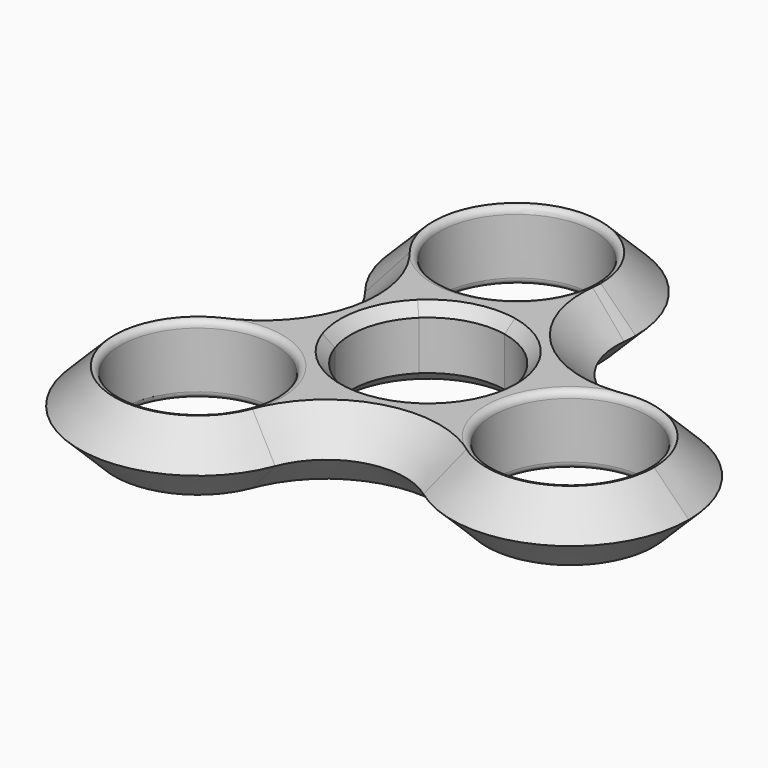
from build123d import *

# Parameters (mm, degrees)
F0_R     = 11.1
F1_DEPTH = 10
F2_SIZE  = 4.99999
F4_SIZE  = 1.5


# Not quite as in the source:
# - a fillet or chamfer that OpenCascade refuses, or shapes differently, is made with other operations: its cross-section is extruded or revolved along the edge and cut away or added
# - a fillet or chamfer is up to 0.001 mm smaller than in the source, because OpenCascade refuses the exact size


with BuildPart() as f1:
    # F0 (on Top) → F1 (new body)
    with BuildSketch(Plane.XY):
        with BuildLine():
            ThreePointArc((-8.9008040787, 8.0483344086), (-3.3470312857, 11.5237746235), (3.2044142943, 11.5642435563))
            ThreePointArc((3.2044142943, 11.5642435563), (7.5784009732, 16.6578149501), (9.6392593011, 23.047579575))
            ThreePointArc((9.6392593011, 23.047579575), (9.7208671752, 24.0063382249), (9.7480988809, 24.9681783508))
            ThreePointArc((9.7480988809, 24.9681783508), (-12.909602396, 40.9990989813), (-20.4860677382, 14.297806572))
            ThreePointArc((-20.4860677382, 14.297806572), (-15.3228623754, 10.0062404951), (-8.9008040787, 8.0483344086))
        make_face()
        with Locations((-7.2519011191, 24.9681783508)):
            Circle(F0_R, mode=Mode.SUBTRACT)
        with BuildLine():
            ThreePointArc((3.2044142943, 11.5642435563), (8.2952723159, 8.6711277931), (11.410994073, 3.7133831296))
            ThreePointArc((11.410994073, 3.7133831296), (16.3058703698, 8.3086431928), (22.5981031738, 10.6504449244))
            ThreePointArc((22.5981031738, 10.6504449244), (13.0446528896, 13.6357009046), (9.6392593011, 23.047579575))
            ThreePointArc((9.6392593011, 23.047579575), (7.5784009732, 16.6578149501), (3.2044142943, 11.5642435563))
        make_face()
        with BuildLine():
            ThreePointArc((22.5981031738, 10.6504449244), (16.3058703698, 8.3086431928), (11.410994073, 3.7133831296))
            ThreePointArc((11.410994073, 3.7133831296), (11.8518338006, 1.8799030726), (12, 0))
            ThreePointArc((12, 0), (11.07283247, -4.6251898438), (8.4346031515, -8.5356587137))
            ThreePointArc((8.4346031515, -8.5356587137), (10.6749837374, -14.8647126588), (15.1909877347, -19.8328045366))
            ThreePointArc((15.1909877347, -19.8328045366), (32.9376604929, -21.3090514083), (42.264828105, -6.139092834))
            ThreePointArc((42.264828105, -6.139092834), (36.302619464, 6.7902212203), (22.5981031738, 10.6504449244))
        make_face()
        with Locations((25.264828105, -6.139092834)):
            Circle(F0_R, mode=Mode.SUBTRACT)
        with BuildLine():
            ThreePointArc((15.1909877347, -19.8328045366), (10.6749837374, -14.8647126588), (8.4346031515, -8.5356587137))
            ThreePointArc((8.4346031515, -8.5356587137), (3.3912632474, -11.5108354861), (-2.459549488, -11.7452380272))
            ThreePointArc((-2.459549488, -11.7452380272), (-1.295062841, -15.2163673164), (-0.9008049677, -18.8563300117))
            ThreePointArc((-0.9008049677, -18.8563300117), (-1.1808473044, -21.9292790409), (-2.0117479955, -24.9009862083))
            ThreePointArc((-2.0117479955, -24.9009862083), (5.3328992991, -18.1012566756), (15.1909877347, -19.8328045366))
        make_face()
        with BuildLine():
            ThreePointArc((-0.9008049677, -18.8563300117), (-1.295062841, -15.2163673164), (-2.459549488, -11.7452380272))
            ThreePointArc((-2.459549488, -11.7452380272), (-8.2619099851, -8.7029215438), (-11.6015857751, -3.0664649849))
            ThreePointArc((-11.6015857751, -3.0664649849), (-18.2060105223, -1.859069951), (-24.7628314098, -3.3027904432))
            ThreePointArc((-24.7628314098, -3.3027904432), (-29.6051774466, -31.1854688655), (-2.0117479955, -24.9009862083))
            ThreePointArc((-2.0117479955, -24.9009862083), (-1.1808473044, -21.9292790409), (-0.9008049677, -18.8563300117))
        make_face()
        with Locations((-17.9008049677, -18.8563300117)):
            Circle(F0_R, mode=Mode.SUBTRACT)
        with BuildLine():
            ThreePointArc((-11.6015857751, -3.0664649849), (-11.6606898946, 2.8334274618), (-8.9008040787, 8.0483344086))
            ThreePointArc((-8.9008040787, 8.0483344086), (-15.3228623754, 10.0062404951), (-20.4860677382, 14.297806572))
            ThreePointArc((-20.4860677382, 14.297806572), (-18.2811908203, 4.4421409517), (-24.7628314098, -3.3027904432))
            ThreePointArc((-24.7628314098, -3.3027904432), (-18.2060105223, -1.859069951), (-11.6015857751, -3.0664649849))
        make_face()
        with BuildLine():
            ThreePointArc((-7.7210685302, 7.9746536446), (-3.0960039393, 10.6594915267), (2.2477068882, 10.8700420305))
            ThreePointArc((2.2477068882, 10.8700420305), (2.732096018, 11.208825126), (3.2044142943, 11.5642435563))
            ThreePointArc((3.2044142943, 11.5642435563), (-3.3470312857, 11.5237746235), (-8.9008040787, 8.0483344086))
            ThreePointArc((-8.9008040787, 8.0483344086), (-8.3115768891, 8.0012373401), (-7.7210685302, 7.9746536446))
        make_face()
        with BuildLine():
            ThreePointArc((-10.5195848427, -3.5423628749), (-10.7861381525, 2.6209204022), (-7.7210685302, 7.9746536446))
            ThreePointArc((-7.7210685302, 7.9746536446), (-8.3115768891, 8.0012373401), (-8.9008040787, 8.0483344086))
            ThreePointArc((-8.9008040787, 8.0483344086), (-11.6606898946, 2.8334274618), (-11.6015857751, -3.0664649849))
            ThreePointArc((-11.6015857751, -3.0664649849), (-11.0564478261, -3.2950069536), (-10.5195848427, -3.5423628749))
        make_face()
        with BuildLine():
            ThreePointArc((2.2477068882, 10.8700420305), (7.6731268923, 8.0207932086), (10.759840528, 2.7268721665))
            ThreePointArc((10.759840528, 2.7268721665), (11.0768405192, 3.2257888132), (11.410994073, 3.7133831296))
            ThreePointArc((11.410994073, 3.7133831296), (8.2952723159, 8.6711277931), (3.2044142943, 11.5642435563))
            ThreePointArc((3.2044142943, 11.5642435563), (2.732096018, 11.208825126), (2.2477068882, 10.8700420305))
        make_face()
        with BuildLine():
            ThreePointArc((10.759840528, 2.7268721665), (11.0146318563, 1.3740033005), (11.1, 0))
            ThreePointArc((11.1, 0), (10.3787556413, -3.9359155654), (8.3087511103, -7.3603434015))
            ThreePointArc((8.3087511103, -7.3603434015), (8.3614588742, -7.9490952222), (8.4346031515, -8.5356587137))
            ThreePointArc((8.4346031515, -8.5356587137), (11.07283247, -4.6251898438), (12, 0))
            ThreePointArc((12, 0), (11.8518338006, 1.8799030726), (11.410994073, 3.7133831296))
            ThreePointArc((11.410994073, 3.7133831296), (11.0768405192, 3.2257888132), (10.759840528, 2.7268721665))
        make_face()
        with BuildLine():
            ThreePointArc((8.4346031515, -8.5356587137), (8.3614588742, -7.9490952222), (8.3087511103, -7.3603434015))
            ThreePointArc((8.3087511103, -7.3603434015), (3.1369185038, -10.6475228246), (-2.9910212262, -10.6894243074))
            ThreePointArc((-2.9910212262, -10.6894243074), (-2.7161060538, -11.2127105225), (-2.459549488, -11.7452380272))
            ThreePointArc((-2.459549488, -11.7452380272), (3.3912632474, -11.5108354861), (8.4346031515, -8.5356587137))
        make_face()
        with BuildLine():
            ThreePointArc((-2.459549488, -11.7452380272), (-2.7161060538, -11.2127105225), (-2.9910212262, -10.6894243074))
            ThreePointArc((-2.9910212262, -10.6894243074), (-7.6422667362, -8.0502024281), (-10.5195848427, -3.5423628749))
            ThreePointArc((-10.5195848427, -3.5423628749), (-11.0564478261, -3.2950069536), (-11.6015857751, -3.0664649849))
            ThreePointArc((-11.6015857751, -3.0664649849), (-8.2619099851, -8.7029215438), (-2.459549488, -11.7452380272))
        make_face()
    extrude(amount=F1_DEPTH)

    # F2 (size 5 in the source; OpenCascade refuses exactly that, so slightly less here)
    f2_edges = [f1.edges().sort_by_distance(p)[0] for p in [
        (-29.605177, -31.185469, 10),
        (41.784139, -10.153115, 0),
    ]]
    chamfer(f2_edges, length=F2_SIZE)

    # F3: fillet of radius 1 on 6 edges, made by hand

    # F3_s1 → F3_t2 (revolve, cut)
    with BuildSketch(Plane.XZ.offset(6.139092834)):
        with BuildLine():
            ThreePointArc((37.364728105, 10.0001), (36.6576213238, 9.7072067812), (36.364728105, 9.0001))
            Line((36.364728105, 9.0001), (36.344728105, 9.0001))
            ThreePointArc((36.344728105, 9.0001), (36.344828105, 9.50005), (36.344828105, 10))
            Line((36.344828105, 10), (36.364828105, 10.02))
            ThreePointArc((36.364828105, 10.02), (36.864778105, 10.02), (37.364728105, 10.0201))
            Line((37.364728105, 10.0201), (37.364728105, 10.0001))
        make_face()
    revolve(axis=Axis((25.264828105, -6.139092834, 10), (0, 0, 1)), mode=Mode.SUBTRACT)

    # F3_s3 → F3_t4 (revolve, cut)
    with BuildSketch(Plane.XZ.offset(-24.9681783508)):
        with BuildLine():
            ThreePointArc((4.8479988809, 10.0001), (4.1408920997, 9.7072067812), (3.8479988809, 9.0001))
            Line((3.8479988809, 9.0001), (3.8279988809, 9.0001))
            ThreePointArc((3.8279988809, 9.0001), (3.8280988809, 9.50005), (3.8280988809, 10))
            Line((3.8280988809, 10), (3.8480988809, 10.02))
            ThreePointArc((3.8480988809, 10.02), (4.3480488809, 10.02), (4.8479988809, 10.0201))
            Line((4.8479988809, 10.0201), (4.8479988809, 10.0001))
        make_face()
    revolve(axis=Axis((-7.2519011191, 24.9681783508, 10), (0, 0, 1)), mode=Mode.SUBTRACT)

    # F3_s5 → F3_t6 (revolve, cut)
    with BuildSketch(Plane.XZ.offset(18.8563300117)):
        with BuildLine():
            ThreePointArc((-5.8009049677, 10.0001), (-6.5080117489, 9.7072067812), (-6.8009049677, 9.0001))
            Line((-6.8009049677, 9.0001), (-6.8209049677, 9.0001))
            ThreePointArc((-6.8209049677, 9.0001), (-6.8208049677, 9.50005), (-6.8208049677, 10))
            Line((-6.8208049677, 10), (-6.8008049677, 10.02))
            ThreePointArc((-6.8008049677, 10.02), (-6.3008549677, 10.02), (-5.8009049677, 10.0201))
            Line((-5.8009049677, 10.0201), (-5.8009049677, 10.0001))
        make_face()
    revolve(axis=Axis((-17.9008049677, -18.8563300117, 10), (0, 0, 1)), mode=Mode.SUBTRACT)

    # F3_s7 → F3_t8 (revolve, cut)
    with BuildSketch(Plane.XZ.offset(6.139092834)):
        with BuildLine():
            ThreePointArc((37.364728105, -0.0001), (36.6576213238, 0.2927932188), (36.364728105, 0.9999))
            Line((36.364728105, 0.9999), (36.344728105, 0.9999))
            ThreePointArc((36.344728105, 0.9999), (36.344828105, 0.49995), (36.344828105, 0))
            Line((36.344828105, 0), (36.364828105, -0.02))
            ThreePointArc((36.364828105, -0.02), (36.864778105, -0.02), (37.364728105, -0.0201))
            Line((37.364728105, -0.0201), (37.364728105, -0.0001))
        make_face()
    revolve(axis=Axis((25.264828105, -6.139092834, 0), (0, 0, 1)), mode=Mode.SUBTRACT)

    # F3_s9 → F3_t10 (revolve, cut)
    with BuildSketch(Plane.XZ.offset(-24.9681783508)):
        with BuildLine():
            ThreePointArc((4.8479988809, -0.0001), (4.1408920997, 0.2927932188), (3.8479988809, 0.9999))
            Line((3.8479988809, 0.9999), (3.8279988809, 0.9999))
            ThreePointArc((3.8279988809, 0.9999), (3.8280988809, 0.49995), (3.8280988809, 0))
            Line((3.8280988809, 0), (3.8480988809, -0.02))
            ThreePointArc((3.8480988809, -0.02), (4.3480488809, -0.02), (4.8479988809, -0.0201))
            Line((4.8479988809, -0.0201), (4.8479988809, -0.0001))
        make_face()
    revolve(axis=Axis((-7.2519011191, 24.9681783508, 0), (0, 0, 1)), mode=Mode.SUBTRACT)

    # F3_s11 → F3_t12 (revolve, cut)
    with BuildSketch(Plane.XZ.offset(18.8563300117)):
        with BuildLine():
            ThreePointArc((-5.8009049677, -0.0001), (-6.5080117489, 0.2927932188), (-6.8009049677, 0.9999))
            Line((-6.8009049677, 0.9999), (-6.8209049677, 0.9999))
            ThreePointArc((-6.8209049677, 0.9999), (-6.8208049677, 0.49995), (-6.8208049677, 0))
            Line((-6.8208049677, 0), (-6.8008049677, -0.02))
            ThreePointArc((-6.8008049677, -0.02), (-6.3008549677, -0.02), (-5.8009049677, -0.0201))
            Line((-5.8009049677, -0.0201), (-5.8009049677, -0.0001))
        make_face()
    revolve(axis=Axis((-17.9008049677, -18.8563300117, 0), (0, 0, 1)), mode=Mode.SUBTRACT)

    # F4
    f4_edges = [f1.edges().sort_by_distance(p)[0] for p in [
        (2.991021, 10.689424, 0),
        (-2.991021, -10.689424, 5),
        (2.991021, 10.689424, 10),
    ]]
    chamfer(f4_edges, length=F4_SIZE)


solid = f1.part
